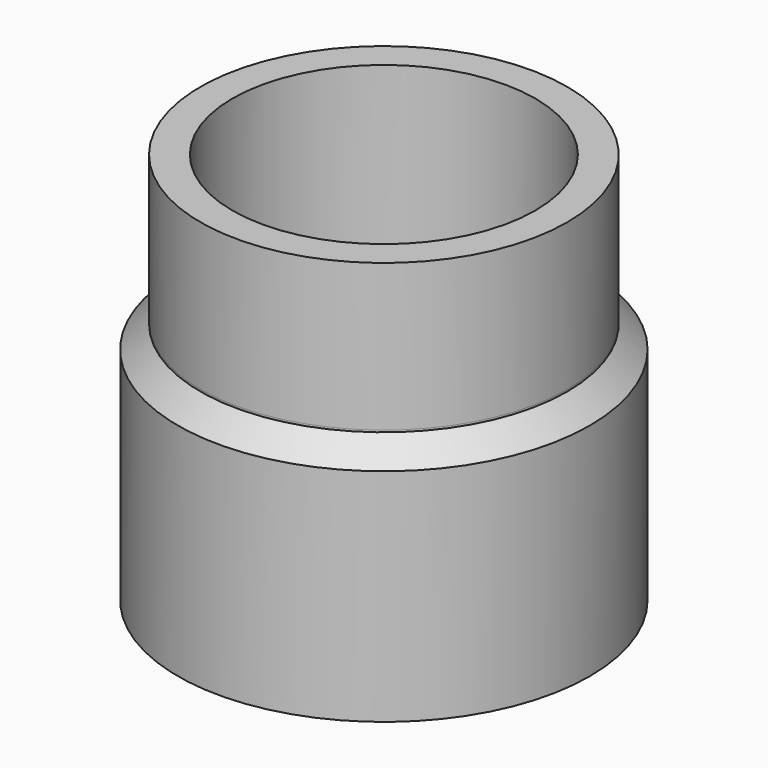
from build123d import *

# Parameters (mm, degrees)
F0_R        = 18.7
F0_R_2      = 15.45
F1_DEPTH    = 20
F0_R_3      = 21
F2_DEPTH    = 5
F3_DEPTH    = 20
F4_S5_R     = 18.7
F4_T6_DEPTH = 31
F5_SIZE     = 3


# Not quite as in the source:
# - a fillet or chamfer that OpenCascade refuses, or shapes differently, is made with other operations: its cross-section is extruded or revolved along the edge and cut away or added


with BuildPart() as f1:
    # F0 (on Top) → F1 (new body)
    with BuildSketch(Plane.XY):
        Circle(F0_R)
        Circle(F0_R_2, mode=Mode.SUBTRACT)
    extrude(amount=F1_DEPTH)

    # F0 (on Top) → F2 (join)
    with BuildSketch(Plane.XY):
        Circle(F0_R_3)
        Circle(F0_R, mode=Mode.SUBTRACT)
    extrude(amount=F2_DEPTH)

    # F0 (on Top) → F3 (join)
    with BuildSketch(Plane.XY):
        Circle(F0_R_3)
        Circle(F0_R, mode=Mode.SUBTRACT)
    extrude(amount=-F3_DEPTH)

    # F4: chamfer of 2.5 on 1 edges, made by hand


with BuildPart() as f4_tool2:
    # F4_s3 → F4_t4 (revolve)
    with BuildSketch(Plane.XZ):
        Polygon((18.5, 5), (21, 2.5), (21, 5), align=None)
    revolve(axis=Axis((0, 0, 5), (0, 0, 1)))

    # F4_s5 → F4_t6 (cut, symmetric)
    with BuildSketch(Plane.XY.offset(3.8)):
        Circle(F4_S5_R)
    extrude(amount=F4_T6_DEPTH, both=True, mode=Mode.SUBTRACT)


with BuildPart() as f1_1:
    add(f1.part)

    # F4_t1: cut F4_tool2
    add(f4_tool2.part, mode=Mode.SUBTRACT)

    # F5
    f5_edges = [f1_1.edges().sort_by_distance(p)[0] for p in [
        (-15.45, 0, 0),
    ]]
    chamfer(f5_edges, length=F5_SIZE)


solid = f1_1.part
